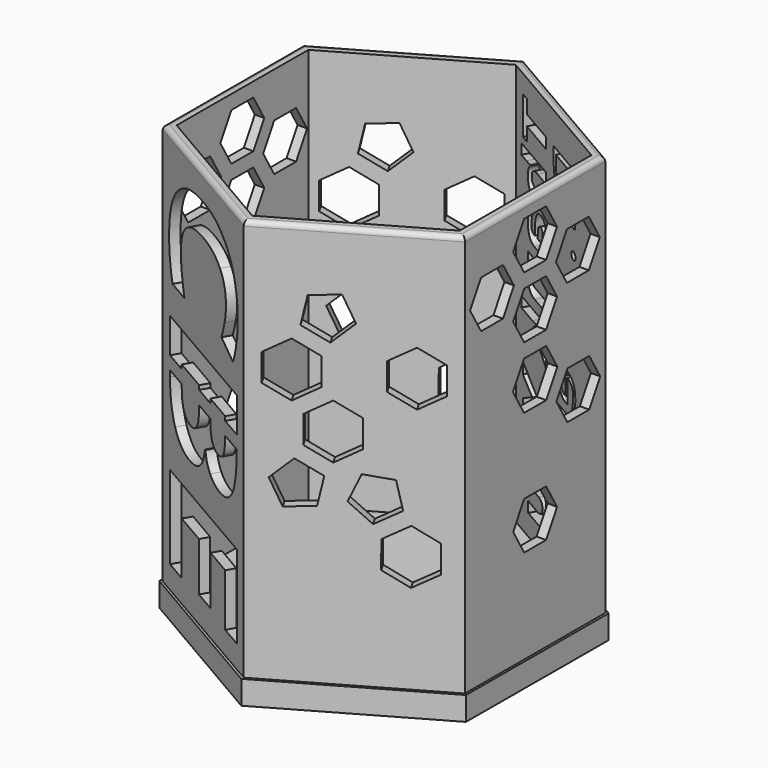
from build123d import *

# Parameters (mm, degrees)
F1_DEPTH      = 90
F3_DEPTH      = 5
F5_DEPTH      = 100
F6_R          = 1
F8_DEPTH      = 100
F10_DEPTH     = 30
F11_TEXT_SIZE = 14.8156941889
F12_TEXT_SIZE = 13.6945898274
F13_DEPTH     = 25
F14_TEXT_SIZE = 2.8591851322
F15_DEPTH     = 2


# Not quite as in the source:
# - Text() gives the source's letters only with a copy of the font that has no kerning and outlines rounded to 1/6400 em; it was checked with that copy


with BuildPart() as f1:
    # F0 (on Top) → F1 (new body)
    with BuildSketch(Plane.XY):
        Polygon((0.088964339, 36.9503101297), (-31.9554250805, 18.5522004425), (-32.0443894195, -18.3981096872), (-0.088964339, -36.9503101297), (31.9554250805, -18.5522004425), (32.0443894195, 18.3981096872), align=None)
        Polygon((-30.0669265299, -17.2040672239), (-29.9326225293, 17.4366885767), (0.1343040006, 34.6407558006), (30.0669265299, 17.2040672239), (29.9326225293, -17.4366885767), (-0.1343040006, -34.6407558006), align=None, mode=Mode.SUBTRACT)
    extrude(amount=F1_DEPTH)

    # F2 (on Top) → F3 (join)
    with BuildSketch(Plane.XY):
        Polygon((32.5707194475, 18.6408574912), (0.141903588, 37.5274992066), (-32.4288158595, 18.8866417154), (-32.5707194475, -18.6408574912), (-0.141903588, -37.5274992066), (32.4288158595, -18.8866417154), align=None)
    extrude(amount=F3_DEPTH)

    # F4 (on face) → F5 (cut)
    with BuildSketch(Plane(origin=(31.99990725, -0.0770453776, 0), x_dir=(0.0024076681, 0.9999971016, 0), z_dir=(0.9999971016, -0.0024076681, 0))):
        Polygon((2.8867513459, 87), (-2.8867513459, 87), (-5.7735026919, 82), (-2.8867513459, 77), (2.8867513459, 77), (5.7735026919, 82), align=None)
        Polygon((14.1450815951, 80.5), (8.3715789032, 80.5), (5.4848275573, 75.5), (8.3715789032, 70.5), (14.1450815951, 70.5), (17.0318329411, 75.5), align=None)
        Polygon((-8.4650974305, 80.6751159435), (-14.2386001224, 80.6751159435), (-17.1253514684, 75.6751159435), (-14.2386001224, 70.6751159435), (-8.4650974305, 70.6751159435), (-5.5783460846, 75.6751159435), align=None)
        Polygon((2.8867513459, 74), (-2.8867513459, 74), (-5.7735026919, 69), (-2.8867513459, 64), (2.8867513459, 64), (5.7735026919, 69), align=None)
        Polygon((-2.9196926255, 61), (-5.839385251, 55.9429440301), (-2.9196926255, 50.8858880602), (2.9196926255, 50.8858880602), (5.839385251, 55.9429440301), (2.9196926255, 61), align=None)
        Polygon((8.4878317097, 54.5301878576), (5.6010803637, 49.5301878576), (8.4878317097, 44.5301878576), (14.2613344016, 44.5301878576), (17.1480857475, 49.5301878576), (14.2613344016, 54.5301878576), align=None)
        Polygon((-2.8867513459, 34.8860689203), (-5.7735026919, 29.8860689203), (-2.8867513459, 24.8860689203), (2.8867513459, 24.8860689203), (5.7735026919, 29.8860689203), (2.8867513459, 34.8860689203), align=None)
    extrude(amount=-F5_DEPTH, mode=Mode.SUBTRACT)

    # F6
    f6_edges = [f1.edges().sort_by_distance(p)[0] for p in [
        (-15.93323, 27.751255, 90),
        (-31.999907, 0.077045, 90),
        (31.999907, -0.077045, 90),
        (15.93323, -27.751255, 90),
        (-16.066677, -27.67421, 90),
        (16.066677, 27.67421, 90),
    ]]
    fillet(f6_edges, radius=F6_R)

    # F7 (on face) → F8 (cut)
    with BuildSketch(Plane(origin=(-15.9332303707, 27.7512552861, 0), x_dir=(-0.8672267277, -0.4979134491, 0), z_dir=(-0.4979134491, 0.8672267277, 0))):
        Polygon((-10.4752086141, 68.7039013911), (-15.4752086141, 65.8171500451), (-15.4752086141, 60.0436473532), (-10.4752086141, 57.1568960073), (-5.4752086141, 60.0436473532), (-5.4752086141, 65.8171500451), align=None)
        Polygon((10.4752086141, 68.7528306789), (5.4752086141, 65.866079333), (5.4752086141, 60.0925766411), (10.4752086141, 57.2058252951), (15.4752086141, 60.0925766411), (15.4752086141, 65.866079333), align=None)
        Polygon((3.5240186518, 57.7549950759), (-1.4759813482, 54.8682437299), (-1.4759813482, 49.094741038), (3.5240186518, 46.2079896921), (8.5240186518, 49.094741038), (8.5240186518, 54.8682437299), align=None)
        Polygon((-9.5219785632, 35.4714362071), (-14.5067950988, 32.5585446129), (-14.4765652476, 26.7851210627), (-9.4615188607, 23.9245891068), (-4.4767023251, 26.837480701), (-4.5069321764, 32.6109042512), align=None)
        Polygon((14.3093467444, 42.6304233792), (10.018798094, 46.4936507362), (5.018798094, 43.6068993903), (6.2191768006, 37.9595615844), (11.9610516407, 37.3560662203), align=None)
        Polygon((-3.1295899867, 35.2789905849), (1.1406721312, 39.1646301434), (-1.235207126, 44.4266194144), (-6.9738433779, 43.7930680739), (-8.1446363736, 38.1395225408), align=None)
        Polygon((2.0612657413, 77.6180852354), (-0.2870293624, 72.3437280765), (4.003519288, 68.4805007195), (9.003519288, 71.3672520655), (7.8031405814, 77.0145898714), align=None)
    extrude(amount=-F8_DEPTH, mode=Mode.SUBTRACT)

    # F9 (on face) → F10 (cut)
    with BuildSketch(Plane(origin=(-16.0666768793, -27.6742099085, 0), x_dir=(0.8648190596, -0.5020836525, 0), z_dir=(-0.5020836525, -0.8648190596, 0))):
        with BuildLine():
            add(Edge.make_bspline(
                [(10.3729953091, 70.2595050061), (10.3729953091, 73.9064755869), (7.6327669567, 75.9066422675)],
                knots=[0, 0, 0, 1, 1, 1], degree=2))
            add(Edge.make_bspline(
                [(9.7696116938, 66.8658888714), (10.3729953091, 68.5926994389), (10.3729953091, 70.2595050061)],
                knots=[0, 0, 0, 1, 1, 1], degree=2))
            add(Edge.make_bspline(
                [(8.3528269617, 63.4256021808), (9.1662280785, 65.1390783038), (9.7696116938, 66.8658888714)],
                knots=[0, 0, 0, 1, 1, 1], degree=2))
            Line((8.3528269617, 63.4256021808), (13.6065981093, 61.345428833))
            add(Edge.make_bspline(
                [(15.7467764575, 70.2595050061), (15.7467764575, 65.8258021975), (13.6065981093, 61.345428833)],
                knots=[0, 0, 0, 1, 1, 1], degree=2))
            add(Edge.make_bspline(
                [(13.8432844998, 77.8534711699), (15.7467764575, 74.6132011474), (15.7467764575, 70.2595050061)],
                knots=[0, 0, 0, 1, 1, 1], degree=2))
            add(Edge.make_bspline(
                [(8.3661614063, 82.8238853711), (11.9397925422, 81.0937411924), (13.8432844998, 77.8534711699)],
                knots=[0, 0, 0, 1, 1, 1], degree=2))
            add(Edge.make_bspline(
                [(0.0388007929, 84.5540295498), (4.7925302703, 84.5540295498), (8.3661614063, 82.8238853711)],
                knots=[0, 0, 0, 1, 1, 1], degree=2))
            add(Edge.make_bspline(
                [(-11.5354970653, 81.033736192), (-7.5018275928, 84.5540295498), (0.0388007929, 84.5540295498)],
                knots=[0, 0, 0, 1, 1, 1], degree=2))
            add(Edge.make_bspline(
                [(-15.5691665377, 70.8662222325), (-15.5691665377, 77.5134428342), (-11.5354970653, 81.033736192)],
                knots=[0, 0, 0, 1, 1, 1], degree=2))
            add(Edge.make_bspline(
                [(-14.0023693046, 62.4921910632), (-15.5691665377, 66.2391699781), (-15.5691665377, 70.8662222325)],
                knots=[0, 0, 0, 1, 1, 1], degree=2))
            Line((-14.0023693046, 62.4921910632), (-8.5885848226, 62.4921910632))
            add(Edge.make_bspline(
                [(-10.188718167, 70.2595050061), (-10.188718167, 67.0525710949), (-8.5885848226, 62.4921910632)],
                knots=[0, 0, 0, 1, 1, 1], degree=2))
            add(Edge.make_bspline(
                [(-0.0012025407, 77.9068089481), (-10.188718167, 77.9068089481), (-10.188718167, 70.2595050061)],
                knots=[0, 0, 0, 1, 1, 1], degree=2))
            add(Edge.make_bspline(
                [(7.6327669567, 75.9066422675), (4.8925386044, 77.9068089481), (-0.0012025407, 77.9068089481)],
                knots=[0, 0, 0, 1, 1, 1], degree=2))
        make_face()
        Polygon((10.0196325288, 49.55111264), (10.0196325288, 48.6693568528), (15.3134070101, 48.6693568528), (15.3134070101, 56.0116510182), (-15.1491315348, 56.0116510182), (-15.1491315348, 48.6693568528), (-9.81535372, 48.6693568528), (-9.81535372, 49.55111264), (-1.8746919982, 49.55111264), (-1.8746919982, 48.6693568528), (3.245734704, 48.6693568528), (3.245734704, 49.55111264), align=None)
        with BuildLine():
            Line((15.3090500038, 45.9091514349), (10.0180712216, 45.9091514349))
            add(Edge.make_bspline(
                [(9.2595691902, 42.1038253661), (9.9851841264, 43.3259136796), (10.0180712216, 45.9091514349)],
                knots=[0, 0, 0, 0.9546769319, 0.9546769319, 0.9546769319], degree=2))
            add(Edge.make_bspline(
                [(6.746026395, 40.8237186905), (8.4995058516, 40.8237186905), (9.2595691902, 42.1038253661)],
                knots=[0, 0, 0, 1, 1, 1], degree=2))
            add(Edge.make_bspline(
                [(4.0591358208, 42.0004834209), (4.8725369375, 40.8237186905), (6.746026395, 40.8237186905)],
                knots=[0, 0, 0, 1, 1, 1], degree=2))
            add(Edge.make_bspline(
                [(3.245734704, 45.8041337251), (3.245734704, 43.1772481513), (4.0591358208, 42.0004834209)],
                knots=[0, 0, 0, 1, 1, 1], degree=2))
            Line((3.245734704, 45.8041337251), (3.245734704, 45.8052046597))
            Line((3.245734704, 45.8052046597), (-1.8746919982, 45.8052046597))
            Line((-1.8746919982, 45.8052046597), (-1.8746919982, 45.5507792789))
            add(Edge.make_bspline(
                [(-5.668341469, 40.1369947969), (-1.8746919982, 40.1369947969), (-1.8746919982, 45.5507792789)],
                knots=[0, 0, 0, 1, 1, 1], degree=2))
            add(Edge.make_bspline(
                [(-8.7952687129, 41.407100639), (-7.7751837058, 40.1369947969), (-5.668341469, 40.1369947969)],
                knots=[0, 0, 0, 1, 1, 1], degree=2))
            add(Edge.make_bspline(
                [(-9.81535372, 45.3440953886), (-9.81535372, 42.6772064812), (-8.7952687129, 41.407100639)],
                knots=[0, 0, 0, 1, 1, 1], degree=2))
            Line((-9.81535372, 45.3440953886), (-9.81535372, 45.9091514349))
            Line((-9.81535372, 45.9091514349), (-15.1491315348, 45.9091514349))
            Line((-15.1491315348, 45.9091514349), (-15.1491315348, 44.6173681613))
            add(Edge.make_bspline(
                [(-12.8156037408, 36.4366864378), (-15.1491315348, 39.4502709032), (-15.1491315348, 44.6173681613)],
                knots=[0, 0, 0, 1, 1, 1], degree=2))
            add(Edge.make_bspline(
                [(-6.315062029, 33.4231019725), (-10.4820759469, 33.4231019725), (-12.8156037408, 36.4366864378)],
                knots=[0, 0, 0, 1, 1, 1], degree=2))
            add(Edge.make_bspline(
                [(-1.6046694963, 34.7065422592), (-3.3748170086, 33.4231019725), (-6.315062029, 33.4231019725)],
                knots=[0, 0, 0, 1, 1, 1], degree=2))
            add(Edge.make_bspline(
                [(0.812198576, 38.8835570104), (0.165478016, 35.9899825459), (-1.6046694963, 34.7065422592)],
                knots=[0, 0, 0, 1, 1, 1], degree=2))
            Line((0.812198576, 38.8835570104), (1.0188824663, 38.8835570104))
            add(Edge.make_bspline(
                [(3.1223910921, 35.4766064312), (1.3722452466, 36.7567131067), (1.0188824663, 38.8835570104)],
                knots=[0, 0, 0, 1, 1, 1], degree=2))
            add(Edge.make_bspline(
                [(7.6060980676, 34.1964997556), (4.8725369375, 34.1964997556), (3.1223910921, 35.4766064312)],
                knots=[0, 0, 0, 1, 1, 1], degree=2))
            add(Edge.make_bspline(
                [(13.4699200528, 37.1234103315), (11.6264330956, 34.1964997556), (7.6060980676, 34.1964997556)],
                knots=[0, 0, 0, 1, 1, 1], degree=2))
            add(Edge.make_bspline(
                [(15.3090500038, 45.9091514349), (15.223785114, 39.9080279151), (13.4699200528, 37.1234103315)],
                knots=[0.0486154218, 0.0486154218, 0.0486154218, 1, 1, 1], degree=2))
        make_face()
        Polygon((-15.1491315348, 27.3425952636), (-15.1491315348, 9.8011334751), (-9.81535372, 9.8011334751), (-9.81535372, 20.8820568854), (-1.9613658877, 20.8820568854), (-1.9613658877, 10.567864036), (3.3324085935, 10.567864036), (3.3324085935, 20.8820568854), (10.0196325288, 20.8820568854), (10.0196325288, 9.8011334751), (15.3134070101, 9.8011334751), (15.3134070101, 27.3425952636), align=None)
    extrude(amount=-F10_DEPTH, mode=Mode.SUBTRACT)

    # F11 (on face) + F12 (on face) → F13 (cut)
    with BuildSketch(Plane(origin=(16.0666768793, 27.6742099085, 0), x_dir=(-0.8648190596, 0.5020836525, 0), z_dir=(0.5020836525, 0.8648190596, 0))):
        with Locations(Location((3.473640442, 86.4436431946), (0, 0, -90))):
            Text('Thank You', F11_TEXT_SIZE, font='Open Sans', font_style=FontStyle.BOLD, text_align=(TextAlign.LEFT, TextAlign.BOTTOM))
    with BuildSketch(Plane(origin=(16.0666768793, 27.6742099085, 0), x_dir=(-0.8648190596, 0.5020836525, 0), z_dir=(0.5020836525, 0.8648190596, 0))):
        with Locations(Location((-9.8601046757, 84.6611589078), (0, 0, -90))):
            Text('Dr. Koelling', F12_TEXT_SIZE, font='Open Sans', text_align=(TextAlign.LEFT, TextAlign.BOTTOM))
    extrude(amount=-F13_DEPTH, mode=Mode.SUBTRACT)

    # F14 (on face) → F15 (cut)
    with BuildSketch(Plane(origin=(0, 0, 0), x_dir=(1, 0, 0), z_dir=(0, 0, -1))):
        with Locations(Location((4.728267148, 1.927800188), (0, 0, -148))):
            Text('LJ.2017', F14_TEXT_SIZE, font='Open Sans', font_style=FontStyle.BOLD, text_align=(TextAlign.LEFT, TextAlign.BOTTOM))
    extrude(amount=-F15_DEPTH, mode=Mode.SUBTRACT)


solid = f1.part
